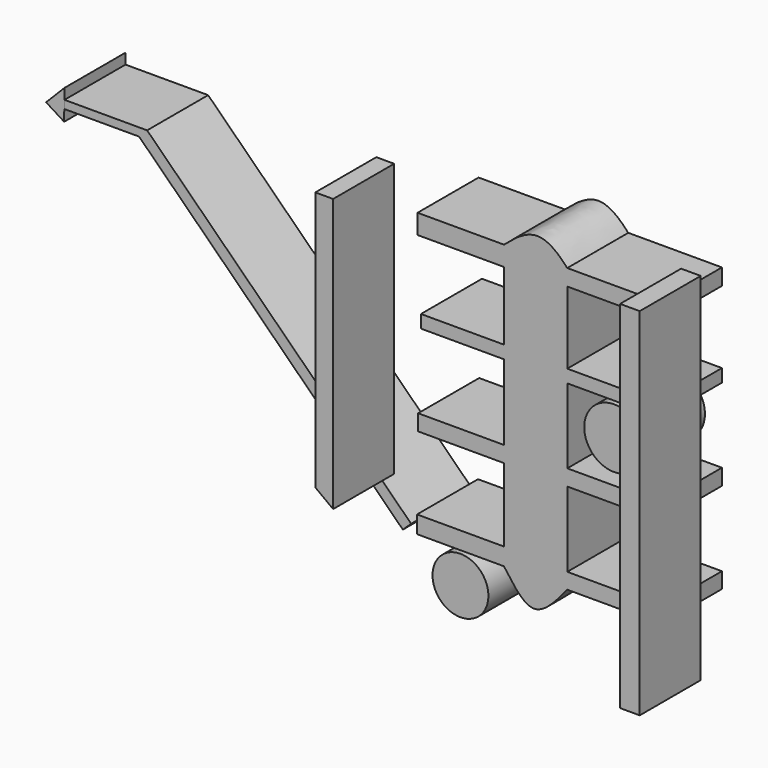
from build123d import *

# Parameters (mm, degrees)
F0_W     = 31.1824278906
F0_H     = 5.4149143398
F0_W_2   = 28.7550520152
F0_H_2   = 6.535243243
F0_W_3   = 27.6347268373
F0_H_3   = 4.2945835739
F0_H_4   = 4.2945872992
F0_H_5   = 5.3215520456
F0_W_4   = 28.5683330148
F0_W_5   = 28.9417747408
F0_H_6   = 5.7883523405
F0_H_7   = 5.2281897515
F1_DEPTH = 25.4
F2_R     = 9.9376162311
F3_DEPTH = 25.4
F2_R_2   = 9.3072509838
F5_DEPTH = 25.4
F4_W     = 5.9344172478
F4_H     = 7.4104368687


# Not quite as in the source:
# - the program builds the solid bodies; features that only make, move or delete a surface that nothing else refers to are left out


with BuildPart() as f1:
    # F0 (on Front) → F1 (new body)
    with BuildSketch(Plane.XZ):
        with Locations((9.9895796739, 56.0163389891)):
            Rectangle(F0_W, F0_H)
        with BuildLine():
            Line((-5.6016342714, 24.9272696674), (-5.6016342714, 29.2218569666))
            Line((-5.6016342714, 29.2218569666), (-5.6016342714, 53.3088818192))
            Line((-5.6016342714, 53.3088818192), (-5.6016342714, 58.723796159))
            add(Edge.make_bspline(
                [(-5.6016342714, 58.723796159), (-5.6426806139, 58.5647439553), (-15.1337303989, 71.2523431637), (-26.5753917973, 58.490990697), (-26.7011206597, 58.723796159)],
                knots=[0, 0, 0, 0, 0.2396480462, 0.4939586428, 0.4939586428, 0.4939586428, 0.4939586428], degree=3))
            Line((-26.7011206597, 58.723796159), (-26.7011206597, 52.188552916))
            Line((-26.7011206597, 52.188552916), (-26.7011206597, 29.408575967))
            Line((-26.7011206597, 29.408575967), (-26.7011206597, 25.113992393))
            Line((-26.7011206597, 25.113992393), (-26.7011206597, 0))
            Line((-26.7011206597, 0), (-26.7011206597, -5.3215520456))
            Line((-26.7011206597, -5.3215520456), (-26.7011206597, -16.7115405202))
            Line((-26.7011206597, -16.7115405202), (-26.7011206597, -29.7820195556))
            Line((-26.7011206597, -29.7820195556), (-26.7011206597, -35.570371896))
            add(Edge.make_bspline(
                [(-26.7011206597, -35.570371896), (-23.4775358451, -40.0920960999), (-16.914419193, -49.2981834607), (-9.4167152022, -40.1998873057), (-5.6016342714, -35.570371896)],
                knots=[0, 0, 0, 0, 0.4911667711, 1, 1, 1, 1], degree=3))
            Line((-5.6016342714, -35.570371896), (-5.6016342714, -30.3421821445))
            Line((-5.6016342714, -30.3421821445), (-5.6016342714, -5.3215520456))
            Line((-5.6016342714, -5.3215520456), (-5.6016342714, 0))
            Line((-5.6016342714, 0), (-5.6016342714, 24.9272696674))
        make_face()
        with Locations((-41.0786466673, 55.4561745375)):
            Rectangle(F0_W_2, F0_H_2)
        with Locations((-40.5184840783, 27.26128418)):
            Rectangle(F0_W_3, F0_H_3)
        with Locations((9.9895796739, 27.074563317)):
            Rectangle(F0_W, F0_H_4)
        with Locations((9.9895796739, -2.6607760228)):
            Rectangle(F0_W, F0_H_5)
        with Locations((-40.9852871671, -2.6607760228)):
            Rectangle(F0_W_4, F0_H_5)
        with Locations((-41.1720080301, -32.6761957258)):
            Rectangle(F0_W_5, F0_H_6)
        with Locations((9.9895796739, -32.9562770203)):
            Rectangle(F0_W, F0_H_7)
    extrude(amount=F1_DEPTH)


with BuildPart() as f3:
    # F2 (on face) → F3 (new body)
    with BuildSketch(Plane.XZ.offset(25.4)):
        with Locations((9.9895796739, 13.9160072431)):
            Circle(F2_R)
    extrude(amount=-F3_DEPTH)


with BuildPart() as f3b:
    # F2 (on face) → F3, piece 2 (new body)
    with BuildSketch(Plane.XZ.offset(25.4)):
        with Locations((-41.1720080301, -45.9239631891)):
            Circle(F2_R_2)
    extrude(amount=-F3_DEPTH)


with BuildPart() as f3c:
    # F2 (on face) → F3, piece 3 (new body)
    with BuildSketch(Plane.XZ.offset(25.4)):
        Polygon((-60.3531059439, -35.778459874), (-57.597335428, -33.1539027393), (-145.5208361149, 53.5896010697), (-148.1922638691, 50.881833114), align=None)
        Polygon((-148.1922638691, 50.881833114), (-145.5208361149, 53.5896010697), (-173.0377972126, 53.5896010697), (-173.0874284987, 50.881833114), align=None)
    extrude(amount=-F3_DEPTH)


with BuildPart() as f3d:
    # F2 (on face) → F3, piece 4 (new body)
    with BuildSketch(Plane.XZ.offset(25.4)):
        Polygon((-173.1564998627, 47.1134595573), (-173.111705617, 50.881833114), (-173.0377972126, 57.0994727314), (-179.1719916159, 50.881833114), align=None)
    extrude(amount=-F3_DEPTH)


with BuildPart() as f5:
    # F4 (on face) → F5 (new body)
    with BuildSketch(Plane.XZ.offset(25.4)):
        Polygon((38.8462878764, 62.9734322429), (32.3033370078, 63.1396621466), (32.3033370078, -47.6440042257), (38.8462878764, -47.6440042257), align=None)
        Polygon((32.3033370078, 70.8710029721), (32.3033370078, 63.1396621466), (38.8462878764, 62.9734322429), (38.8462878764, 70.8710029721), align=None)
    extrude(amount=F5_DEPTH)


with BuildPart() as f5b:
    # F4 (on face) → F5, piece 2 (new body)
    with BuildSketch(Plane.XZ.offset(25.4)):
        with Locations((-66.2259534001, 66.8448805809)):
            Rectangle(F4_W, F4_H)
        Polygon((-63.2587447762, -20.3745421022), (-63.2587447762, 63.1396621466), (-69.193162024, 63.1396621466), (-69.193162024, -15.9559678286), align=None)
    extrude(amount=F5_DEPTH)


solid = Compound([f1.part, f3.part, f3b.part, f3c.part, f3d.part, f5.part, f5b.part])
